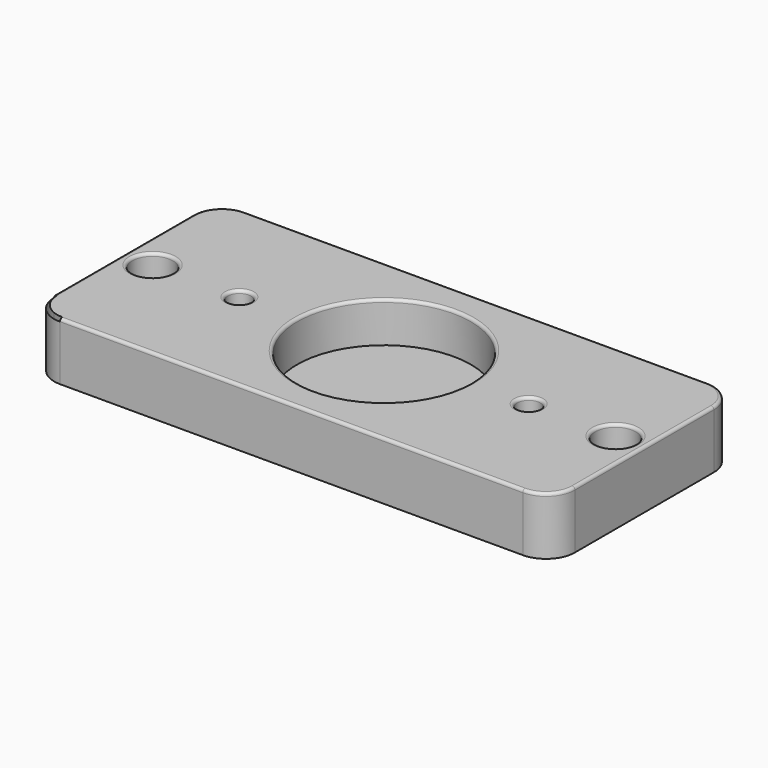
from build123d import *

# Parameters (mm, degrees)
F0_W         = 90
F0_H         = 40
F0_R         = 3.5
F0_R_2       = 2
F1_DEPTH     = 10
F2_R         = 15
F3_DEPTH     = 7
F4_R         = 0.5
F5_T1_DEPTH  = 22.5
F5_T4_ANGLE  = 90
F5_T6_ANGLE  = 90
F5_T8_ANGLE  = 90
F5_T10_ANGLE = 90


# Not quite as in the source:
# - a fillet or chamfer that OpenCascade refuses, or shapes differently, is made with other operations: its cross-section is extruded or revolved along the edge and cut away or added
# - a feature names something its author has since deleted; it is built from what else it names


with BuildPart() as f1:
    # F0 (on Top) → F1 (new body)
    with BuildSketch(Plane.XY):
        Rectangle(F0_W, F0_H)
        with Locations((-40, 0)):
            Circle(F0_R, mode=Mode.SUBTRACT)
        with Locations((-25, 0)):
            Circle(F0_R_2, mode=Mode.SUBTRACT)
        with Locations((25, 0)):
            Circle(F0_R_2, mode=Mode.SUBTRACT)
        with Locations((40, 0)):
            Circle(F0_R, mode=Mode.SUBTRACT)
    extrude(amount=F1_DEPTH)

    # F2 (on face) → F3 (cut)
    with BuildSketch(Plane.XY.offset(10)):
        Circle(F2_R)
    extrude(amount=-F3_DEPTH, mode=Mode.SUBTRACT)

    # F4
    f4_edges = [f1.edges().sort_by_distance(p)[0] for p in [
        (0, -20, 10),
        (-45, 0, 10),
        (45, 0, 10),
        (0, 20, 10),
        (-43.5, 0, 10),
        (-27, 0, 10),
        (-15, 0, 10),
        (23, 0, 10),
        (36.5, 0, 10),
    ]]
    fillet(f4_edges, radius=F4_R)

    # F5: fillet of radius 5 on 4 edges, made by hand

    # F5_s2 → F5_t1 (cut)
    with BuildSketch(Plane.XY.offset(-12.5)):
        with BuildLine():
            ThreePointArc((40, -20), (43.5355339059, -18.5355339059), (45, -15))
            Line((45, -15), (45, -20))
            Line((45, -20), (40, -20))
        make_face()
        with BuildLine():
            ThreePointArc((-40, -20), (-43.5355339059, -18.5355339059), (-45, -15))
            Line((-45, -15), (-45, -20))
            Line((-45, -20), (-40, -20))
        make_face()
        with BuildLine():
            ThreePointArc((45, 15), (43.5355339059, 18.5355339059), (40, 20))
            Line((40, 20), (45, 20))
            Line((45, 20), (45, 15))
        make_face()
        with BuildLine():
            ThreePointArc((-45, 15), (-43.5355339059, 18.5355339059), (-40, 20))
            Line((-40, 20), (-45, 20))
            Line((-45, 20), (-45, 15))
        make_face()
    extrude(amount=F5_T1_DEPTH, mode=Mode.SUBTRACT)

    # F5_s3 → F5_t4 (revolve, cut)
    with BuildSketch(Plane.YZ.offset(-40)):
        with BuildLine():
            ThreePointArc((19.5, 10), (19.8535533906, 9.8535533906), (20, 9.5))
            Line((20, 9.5), (20, 10))
            Line((20, 10), (19.5, 10))
        make_face()
    revolve(axis=Axis((-40, 15, 10), (0, 0, 1)), revolution_arc=F5_T4_ANGLE, mode=Mode.SUBTRACT)

    # F5_s5 → F5_t6 (revolve, cut)
    with BuildSketch(Plane.XZ.offset(-15)):
        with BuildLine():
            ThreePointArc((44.5, 10), (44.8535533906, 9.8535533906), (45, 9.5))
            Line((45, 9.5), (45, 10))
            Line((45, 10), (44.5, 10))
        make_face()
    revolve(axis=Axis((40, 15, 10), (0, 0, 1)), revolution_arc=F5_T6_ANGLE, mode=Mode.SUBTRACT)

    # F5_s7 → F5_t8 (revolve, cut)
    with BuildSketch(Plane.XZ.offset(15)):
        with BuildLine():
            ThreePointArc((-44.5, 10), (-44.8535533906, 9.8535533906), (-45, 9.5))
            Line((-45, 9.5), (-45, 10))
            Line((-45, 10), (-44.5, 10))
        make_face()
    revolve(axis=Axis((-40, -15, 10), (0, 0, 1)), revolution_arc=F5_T8_ANGLE, mode=Mode.SUBTRACT)

    # F5_s9 → F5_t10 (revolve, cut)
    with BuildSketch(Plane.YZ.offset(40)):
        with BuildLine():
            ThreePointArc((-19.5, 10), (-19.8535533906, 9.8535533906), (-20, 9.5))
            Line((-20, 9.5), (-20, 10))
            Line((-20, 10), (-19.5, 10))
        make_face()
    revolve(axis=Axis((40, -15, 10), (0, 0, 1)), revolution_arc=F5_T10_ANGLE, mode=Mode.SUBTRACT)


solid = f1.part
